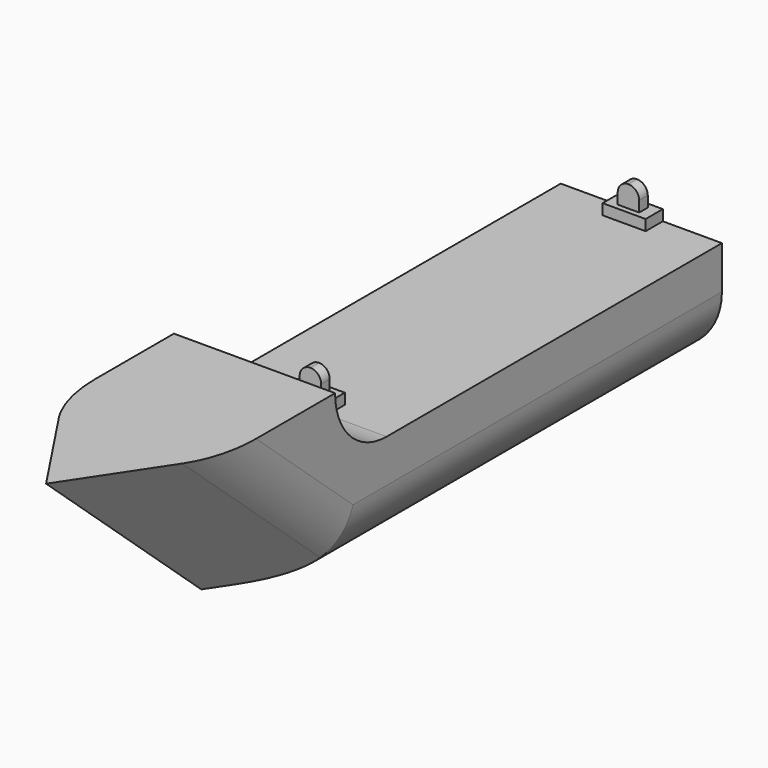
from build123d import *

# Parameters (mm, degrees)
F1_DEPTH    = 19.05
F2_T1_DEPTH = 82.895018686
F3_R        = 7.61999
F5_W        = 2.54
F5_H        = 1.27
F6_DEPTH    = 3.81
F4_W        = 5.08
F4_H        = 2.54
F7_DEPTH    = 1.27
F8_R        = 1.26999


# Not quite as in the source:
# - a fillet or chamfer that OpenCascade refuses, or shapes differently, is made with other operations: its cross-section is extruded or revolved along the edge and cut away or added
# - a fillet or chamfer is up to 0.001 mm smaller than in the source, because OpenCascade refuses the exact size


with BuildPart() as f1:
    # F0 (on Right) → F1 (new body)
    with BuildSketch(Plane.YZ):
        Polygon((-22.9305560945, 20.32), (0, 0), (65.9694439055, 0), (65.9694439055, 12.7), (8.8194439055, 12.7), (8.8194439055, 20.32), align=None)
    extrude(amount=F1_DEPTH)

    # F2: chamfer of 10.16 on 2 edges, made by hand

    # F2_s2 → F2_t1 (cut)
    with BuildSketch(Plane(origin=(0, -42.4856252608, 37.6487993462), x_dir=(1, 0, 0), z_dir=(0, 0.7484248802, -0.6632195705))):
        Polygon((8.89, 0), (19.05, -10.16), (19.05, 0), align=None)
        Polygon((10.16, 0), (0, -10.16), (0, 0), align=None)
    extrude(amount=F2_T1_DEPTH, mode=Mode.SUBTRACT)

    # F3 (radius 7.62 in the source; OpenCascade refuses exactly that, so slightly less here)
    f3_edges = [f1.edges().sort_by_distance(p)[0] for p in [
        (0, 3.853932, 10.16),
        (0, 40.644327, 0),
        (19.05, 40.644327, 0),
        (19.05, 3.853932, 10.16),
        (9.525, 8.819444, 12.7),
    ]]
    fillet(f3_edges, radius=F3_R)

    # F5 (on face) → F6 (join)
    with BuildSketch(Plane.XY.offset(12.7)):
        with Locations((9.525, 17.7094439055)):
            Rectangle(F5_W, F5_H)
        with Locations((9.525, 64.6994439055)):
            Rectangle(F5_W, F5_H)
    extrude(amount=F6_DEPTH)

    # F4 (on face) → F7 (join)
    with BuildSketch(Plane.XY.offset(12.7)):
        with Locations((9.525, 17.7094439055)):
            Rectangle(F4_W, F4_H)
        with Locations((9.525, 64.6994439055)):
            Rectangle(F4_W, F4_H)
    extrude(amount=F7_DEPTH)

    # F8 (radius 1.27 in the source; OpenCascade refuses exactly that, so slightly less here)
    f8_edges = [f1.edges().sort_by_distance(p)[0] for p in [
        (10.795, 17.709444, 16.51),
        (8.255, 17.709444, 16.51),
        (8.255, 64.699444, 16.51),
        (10.795, 64.699444, 16.51),
    ]]
    fillet(f8_edges, radius=F8_R)


solid = f1.part
